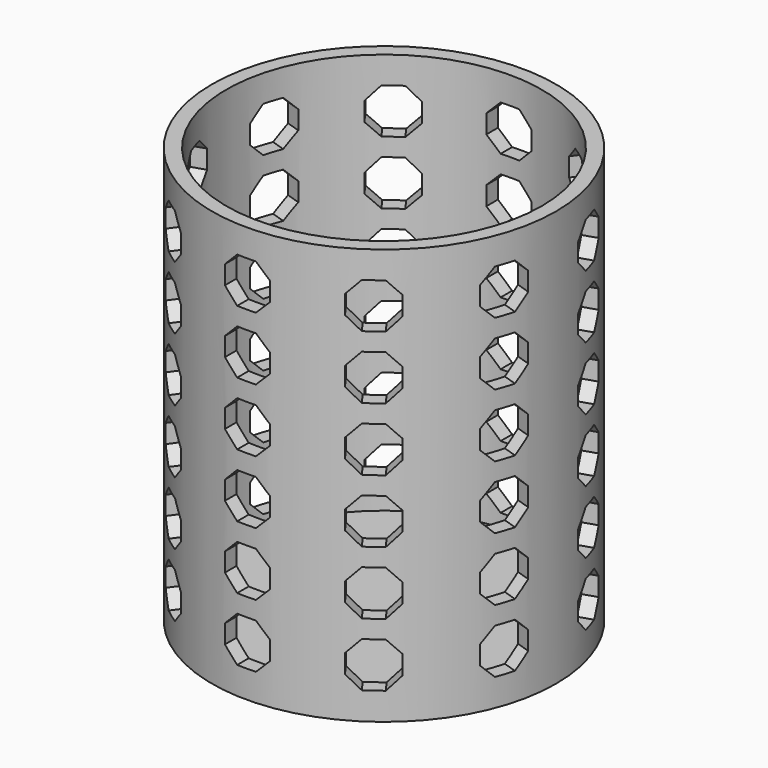
from build123d import *

# Parameters (mm, degrees)
F0_R            = 38.1
F1_DEPTH        = 3.175
F2_R            = 38.1
F2_R_2          = 34.925
F3_DEPTH        = 88.9
F6_DEPTH        = 38.101
F6_COPIES_COUNT = 10


# Not quite as in the source:
# - a pattern or mirror of a feature is missing from the dataset's text; its kind, count and spacing are read off the source's solid


with BuildPart() as f1:
    # F0 (on Top) → F1 (new body)
    with BuildSketch(Plane.XY):
        Circle(F0_R)
    extrude(amount=F1_DEPTH)

    # F2 (on face) → F3 (join)
    with BuildSketch(Plane.XY.offset(3.175)):
        Circle(F2_R)
        Circle(F2_R_2, mode=Mode.SUBTRACT)
    extrude(amount=F3_DEPTH)

    # F5 (on Front) → F6 (cut, through all)
    with BuildSketch(Plane.XZ):
        Polygon((5, 83.1460678119), (2.0710678119, 86.075), (-2.0710678119, 86.075), (-5, 83.1460678119), (-5, 79.0039321881), (-2.0710678119, 76.075), (2.0710678119, 76.075), (5, 79.0039321881), align=None)
        Polygon((2.0710678119, 72.075), (-2.0710678119, 72.075), (-5, 69.1460678119), (-5, 65.0039321881), (-2.0710678119, 62.075), (2.0710678119, 62.075), (5, 65.0039321881), (5, 69.1460678119), align=None)
        Polygon((2.0710678119, 58.075), (-2.0710678119, 58.075), (-5, 55.1460678119), (-5, 51.0039321881), (-2.0710678119, 48.075), (2.0710678119, 48.075), (5, 51.0039321881), (5, 55.1460678119), align=None)
        Polygon((2.0710678119, 44.075), (-2.0710678119, 44.075), (-5, 41.1460678119), (-5, 37.0039321881), (-2.0710678119, 34.075), (2.0710678119, 34.075), (5, 37.0039321881), (5, 41.1460678119), align=None)
        Polygon((2.0710678119, 30.075), (-2.0710678119, 30.075), (-5, 27.1460678119), (-5, 23.0039321881), (-2.0710678119, 20.075), (2.0710678119, 20.075), (5, 23.0039321881), (5, 27.1460678119), align=None)
        Polygon((2.0710678119, 16.075), (-2.0710678119, 16.075), (-5, 13.1460678119), (-5, 9.0039321881), (-2.0710678119, 6.075), (2.0710678119, 6.075), (5, 9.0039321881), (5, 13.1460678119), align=None)
    f6 = extrude(amount=-F6_DEPTH, mode=Mode.SUBTRACT)

    # F6_copies: F6 ×10 about axis
    f6_copies_axis = Axis((0, 0, 0), (0, 0, 1))
    for i in range(1, F6_COPIES_COUNT):
        add(f6.rotate(f6_copies_axis, i * 360 / F6_COPIES_COUNT), mode=Mode.SUBTRACT)


solid = f1.part
